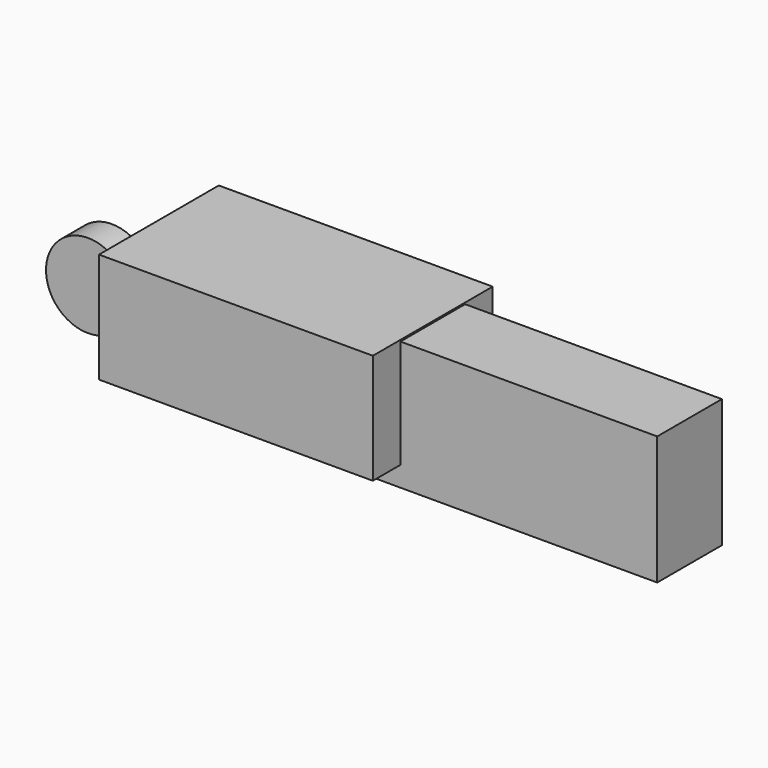
from build123d import *

# Parameters (mm, degrees)
F0_W     = 46.4502461255
F0_H     = 18.6690017581
F3_DEPTH = 12.7
F4_DEPTH = 12.7
F1_R     = 7.1154754627
F5_DEPTH = 2.54
F6_DEPTH = 2.54
F2_W     = 69.1488236189
F2_H     = 21.8198187649
F7_DEPTH = 6.858
F8_DEPTH = 6.858


# Not quite as in the source:
# - the program builds the solid bodies; features that only make, move or delete a surface that nothing else refers to are left out


with BuildPart() as f3:
    # F0 (on Front) → F3 (new body)
    with BuildSketch(Plane.XZ):
        with Locations((-66.7861234397, -63.1189979613)):
            Rectangle(F0_W, F0_H)
    extrude(amount=F3_DEPTH)

    # F4 (add): a face of the model
    f4_faces = [f3.faces().sort_by_distance(p)[0] for p in [
        (-66.7861234397, 0, -63.1189979613),
    ]]
    extrude(f4_faces, amount=F4_DEPTH)

    # F2 (on Front) → F7 (join)
    with BuildSketch(Plane.XZ):
        with Locations((-34.5744118094, -64.9482440203)):
            Rectangle(F2_W, F2_H)
    extrude(amount=F7_DEPTH)

    # F8 (add): a face of the model
    f8_faces = [f3.faces().sort_by_distance(p)[0] for p in [
        (-24.68336426, 0, -65.7213116697),
    ]]
    extrude(f8_faces, amount=F8_DEPTH)


with BuildPart() as f5:
    # F1 (on Front) → F5 (new body)
    with BuildSketch(Plane.XZ):
        with Locations((-100.0125035644, -65.7860040665)):
            Circle(F1_R)
    extrude(amount=F5_DEPTH)

    # F6 (add): a face of the model
    f6_faces = [f5.faces().sort_by_distance(p)[0] for p in [
        (-100.0125035644, 0, -65.7860040665),
    ]]
    extrude(f6_faces, amount=F6_DEPTH)


solid = Compound([f3.part, f5.part])
